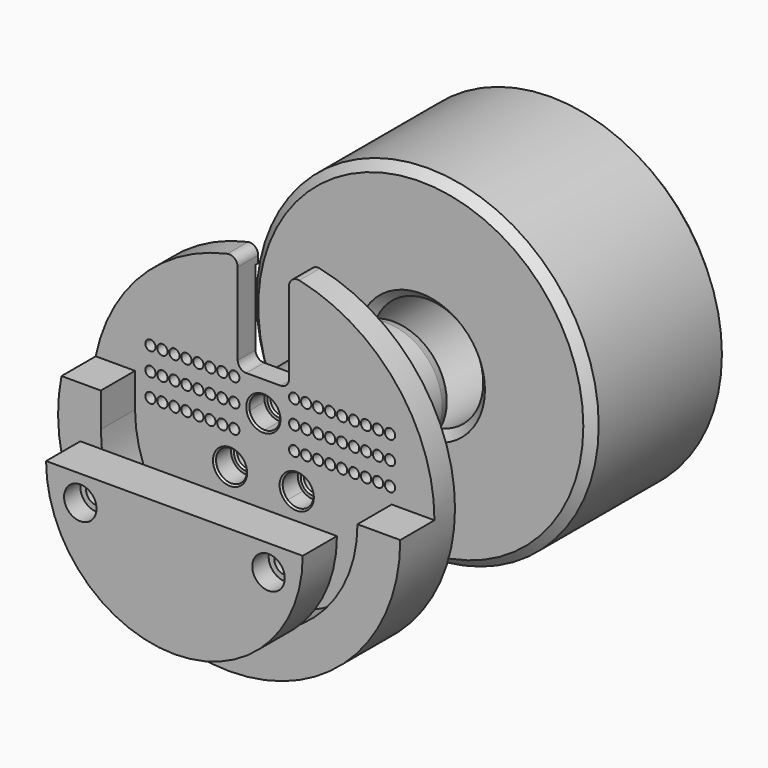
from build123d import *

# Parameters (mm, degrees)
F0_R      = 100
F0_R_2    = 32.5
F1_DEPTH  = 100
F2_SIZE   = 5
F4_R      = 32.5
F5_DEPTH  = 80
F6_SIZE2  = 1.3397459622
F6_SIZE   = 5
F7_R      = 100
F8_DEPTH  = 15
F9_R      = 90
F9_R_2    = 32.5
F10_DEPTH = 2
F11_W     = 15
F11_H     = 60
F12_DEPTH = 25
F13_R     = 5
F15_DEPTH = 12
F16_R     = 6.25
F17_DEPTH = 25
F18_SIZE  = 1
F20_DEPTH = 25
F23_DEPTH = 25
F24_R     = 9.5
F24_R_2   = 6.25
F25_DEPTH = 12
F26_R     = 6.25
F27_DEPTH = 15
F28_R     = 3
F29_DEPTH = 10


# Not quite as in the source:
# - a feature names something its author has since deleted; it is built from what else it names


with BuildPart() as f1:
    # F0 (on Front) → F1 (new body)
    with BuildSketch(Plane.XZ):
        Circle(F0_R)
        Circle(F0_R_2, mode=Mode.SUBTRACT)
    extrude(amount=F1_DEPTH)

    # F2
    f2_edges = [f1.edges().sort_by_distance(p)[0] for p in [
        (-32.5, -100, 0),
        (-100, -100, 0),
        (-100, 0, 0),
        (-32.5, 0, 0),
    ]]
    chamfer(f2_edges, length=F2_SIZE)


with BuildPart() as f5:
    # F4 (on offset) → F5 (new body)
    with BuildSketch(Plane.XZ.offset(200)):
        Circle(F4_R)
    extrude(amount=-F5_DEPTH)

    # F6
    f6_edges = [f5.edges().sort_by_distance(p)[0] for p in [
        (-32.5, -120, 0),
    ]]
    f6_side = f5.faces().sort_by_distance((-32.5, -160, 0))[0]
    chamfer(f6_edges, length=F6_SIZE, length2=F6_SIZE2, reference=f6_side)

    # F7 (on face) → F8 (join)
    with BuildSketch(Plane.XZ.offset(200)):
        Circle(F7_R)
    extrude(amount=F8_DEPTH)

    # F9 (on face) → F10 (cut)
    with BuildSketch(Plane(origin=(0, -200, 0), x_dir=(-1, 0, 0), z_dir=(0, 1, 0))):
        Circle(F9_R)
        Circle(F9_R_2, mode=Mode.SUBTRACT)
    extrude(amount=-F10_DEPTH, mode=Mode.SUBTRACT)

    # F11 (on face) → F12 (cut)
    with BuildSketch(Plane(origin=(0, -200, 0), x_dir=(-1, 0, 0), z_dir=(0, 1, 0))):
        with Locations((-7.5, 70)):
            Rectangle(F11_W, F11_H)
        with Locations((7.5, 70)):
            Rectangle(F11_W, F11_H)
    extrude(amount=-F12_DEPTH, mode=Mode.SUBTRACT)

    # F13
    f13_edges = [f5.edges().sort_by_distance(p)[0] for p in [
        (-15, -208.5, 40),
        (15, -208.5, 40),
        (15, -207.5, 98.8686),
        (-15, -207.5, 98.8686),
    ]]
    fillet(f13_edges, radius=F13_R)

    # F14 (on face) → F15 (cut)
    with BuildSketch(Plane.XZ.offset(215)):
        with BuildLine():
            Line((0, 13.5), (0, 22.5))
            ThreePointArc((0, 22.5), (-4.5, 22.045407685), (-8.818163074, 20.7))
            ThreePointArc((-8.818163074, 20.7), (-5.6920997883, 15.5286299768), (0, 13.5))
        make_face()
        with BuildLine():
            ThreePointArc((0, 13.5), (5.6920997883, 15.5286299768), (8.818163074, 20.7))
            ThreePointArc((8.818163074, 20.7), (4.5, 22.045407685), (0, 22.5))
            Line((0, 22.5), (0, 13.5))
        make_face()
        with BuildLine():
            ThreePointArc((0, 22.5), (4.5, 22.045407685), (8.818163074, 20.7))
            ThreePointArc((8.818163074, 20.7), (8.954425377, 21.595419342), (9, 22.5))
            ThreePointArc((9, 22.5), (6.3639610242, 28.8639610372), (-1.84e-08, 31.5))
            ThreePointArc((-1.84e-08, 31.5), (-6.971370029, 28.1920997812), (-8.818163074, 20.7))
            ThreePointArc((-8.818163074, 20.7), (-4.5, 22.045407685), (0, 22.5))
        make_face()
        with BuildLine():
            ThreePointArc((-22.3358073953, -2.7132467632), (-19.4855715851, -11.25), (-13.5176443213, -17.9867532368))
            ThreePointArc((-13.5176443213, -17.9867532368), (-11.2785214033, -14.9438228589), (-10.4855715851, -11.25))
            ThreePointArc((-10.4855715851, -11.25), (-14.224969067, -3.9475304762), (-22.3358073953, -2.7132467632))
        make_face()
        with BuildLine():
            ThreePointArc((-27.2798001221, -15.7500001682), (-20.9293894952, -20.133433449), (-13.5176443213, -17.9867532368))
            ThreePointArc((-13.5176443213, -17.9867532368), (-19.4855715851, -11.25), (-22.3358073953, -2.7132467632))
            ThreePointArc((-22.3358073953, -2.7132467632), (-27.9007596487, -8.0586664457), (-27.2798001221, -15.7500001682))
        make_face()
        with BuildLine():
            ThreePointArc((28.4855715851, -11.25), (26.7880411089, -5.9893974818), (22.3358073953, -2.7132467632))
            ThreePointArc((22.3358073953, -2.7132467632), (19.4855715851, -11.25), (13.5176443213, -17.9867532368))
            ThreePointArc((13.5176443213, -17.9867532368), (20.9293894839, -20.1334334508), (27.2798001106, -15.750000188))
            ThreePointArc((27.2798001106, -15.750000188), (28.1789039937, -13.5793715108), (28.4855715851, -11.25))
        make_face()
        with BuildLine():
            ThreePointArc((13.5176443213, -17.9867532368), (19.4855715851, -11.25), (22.3358073953, -2.7132467632))
            ThreePointArc((22.3358073953, -2.7132467632), (11.6913429511, -6.75), (13.5176443213, -17.9867532368))
        make_face()
    extrude(amount=-F15_DEPTH, mode=Mode.SUBTRACT)

    # F16 (on face) → F17 (cut)
    with BuildSketch(Plane.XZ.offset(203)):
        with Locations((0, 22.5)):
            Circle(F16_R)
        with Locations((19.4855715851, -11.25)):
            Circle(F16_R)
        with Locations((-19.4855715851, -11.25)):
            Circle(F16_R)
    extrude(amount=-F17_DEPTH, mode=Mode.SUBTRACT)

    # F18
    f18_edges = [f5.edges().sort_by_distance(p)[0] for p in [
        (-8.818163, -215, 24.3),
        (-6.25, -203, 22.5),
        (16.635336, -215, -19.786753),
        (13.235572, -203, -11.25),
        (-25.735572, -203, -11.25),
        (-16.635336, -215, -19.786753),
    ]]
    chamfer(f18_edges, length=F18_SIZE)

    # F19 (on face) → F20 (join)
    with BuildSketch(Plane.XZ.offset(215)):
        with BuildLine():
            ThreePointArc((75, 0), (0, -75), (-75, 0))
            Line((-75, 0), (-75, 20))
            Line((-75, 20), (-97.9795897113, 20))
            ThreePointArc((-97.9795897113, 20), (-10.0508962005, -99.4936153005), (100, 0))
            Line((100, 0), (75, 0))
        make_face()
    extrude(amount=F20_DEPTH)

    # F28 (on face) → F29 (cut)
    with BuildSketch(Plane.XZ.offset(215)):
        with Locations((74, 9)):
            Circle(F28_R)
        with Locations((67, 9)):
            Circle(F28_R)
        with Locations((60, 9)):
            Circle(F28_R)
        with Locations((53, 9)):
            Circle(F28_R)
        with Locations((46, 9)):
            Circle(F28_R)
        with Locations((39, 9)):
            Circle(F28_R)
        with Locations((32, 9)):
            Circle(F28_R)
        with Locations((25, 9)):
            Circle(F28_R)
        with Locations((18, 9)):
            Circle(F28_R)
        with Locations((-17, 9)):
            Circle(F28_R)
        with Locations((-24, 9)):
            Circle(F28_R)
        with Locations((-31, 9)):
            Circle(F28_R)
        with Locations((-38, 9)):
            Circle(F28_R)
        with Locations((74, 36)):
            Circle(F28_R)
        with Locations((67, 36)):
            Circle(F28_R)
        with Locations((60, 36)):
            Circle(F28_R)
        with Locations((53, 36)):
            Circle(F28_R)
        with Locations((39, 36)):
            Circle(F28_R)
        with Locations((32, 36)):
            Circle(F28_R)
        with Locations((25, 36)):
            Circle(F28_R)
        with Locations((-17, 36)):
            Circle(F28_R)
        with Locations((-45, 9)):
            Circle(F28_R)
        with Locations((-52, 9)):
            Circle(F28_R)
        with Locations((-59, 36)):
            Circle(F28_R)
        with Locations((-38, 36)):
            Circle(F28_R)
        with Locations((-31, 36)):
            Circle(F28_R)
        with Locations((46, 36)):
            Circle(F28_R)
        with Locations((18, 36)):
            Circle(F28_R)
        with Locations((-24, 36)):
            Circle(F28_R)
        with Locations((-52, 36)):
            Circle(F28_R)
        with Locations((-66, 36)):
            Circle(F28_R)
        with Locations((-45, 36)):
            Circle(F28_R)
        with Locations((-59, 9)):
            Circle(F28_R)
        with Locations((-66, 9)):
            Circle(F28_R)
        with Locations((-52, 22.5)):
            Circle(F28_R)
        with Locations((-45, 22.5)):
            Circle(F28_R)
        with Locations((-38, 22.5)):
            Circle(F28_R)
        with Locations((-31, 22.5)):
            Circle(F28_R)
        with Locations((-24, 22.5)):
            Circle(F28_R)
        with Locations((-17, 22.5)):
            Circle(F28_R)
        with Locations((18, 22.5)):
            Circle(F28_R)
        with Locations((25, 22.5)):
            Circle(F28_R)
        with Locations((32, 22.5)):
            Circle(F28_R)
        with Locations((39, 22.5)):
            Circle(F28_R)
        with Locations((46, 22.5)):
            Circle(F28_R)
        with Locations((53, 22.5)):
            Circle(F28_R)
        with Locations((60, 22.5)):
            Circle(F28_R)
        with Locations((67, 22.5)):
            Circle(F28_R)
        with Locations((74, 22.5)):
            Circle(F28_R)
        with Locations((-59, 22.5)):
            Circle(F28_R)
        with Locations((-66, 22.5)):
            Circle(F28_R)
    extrude(amount=-F29_DEPTH, mode=Mode.SUBTRACT)


with BuildPart() as f23:
    # F22 (on offset) → F23 (new body)
    with BuildSketch(Plane.XZ.offset(255)):
        with BuildLine():
            Line((75, 0), (-75, 0))
            ThreePointArc((-75, 0), (0, -75), (75, 0))
        make_face()
    extrude(amount=F23_DEPTH)

    # F24 (on face) → F25 (cut)
    with BuildSketch(Plane.XZ.offset(280)):
        with Locations((-55, -15)):
            Circle(F24_R)
        with Locations((-55, -15)):
            Circle(F24_R_2, mode=Mode.SUBTRACT)
        with Locations((55, -15)):
            Circle(F24_R)
        with Locations((55, -15)):
            Circle(F24_R_2, mode=Mode.SUBTRACT)
        with Locations((-55, -15)):
            Circle(F24_R_2)
        with Locations((55, -15)):
            Circle(F24_R_2)
    extrude(amount=-F25_DEPTH, mode=Mode.SUBTRACT)

    # F26 (on face) → F27 (cut)
    with BuildSketch(Plane.XZ.offset(268)):
        with Locations((-55, -15)):
            Circle(F26_R)
        with Locations((55, -15)):
            Circle(F26_R)
    extrude(amount=-F27_DEPTH, mode=Mode.SUBTRACT)


solid = Compound([f1.part, f5.part, f23.part])
